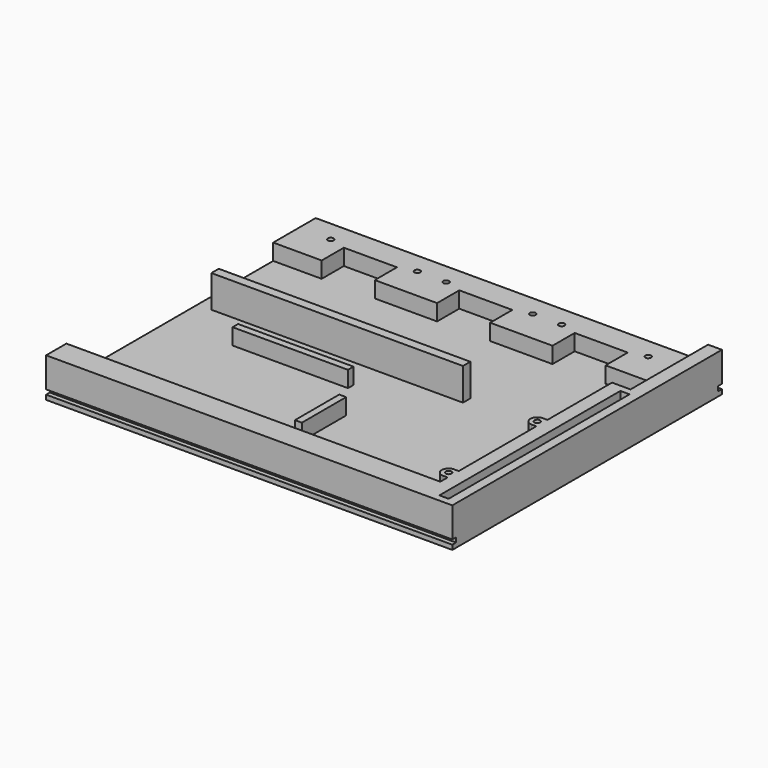
from build123d import *

# Parameters (mm, degrees)
F0_W      = 176
F0_H      = 146
F1_DEPTH  = 3
F2_W      = 50
F2_H      = 3
F2_W_2    = 3
F2_H_2    = 24
F2_W_3    = 109
F2_H_3    = 4
F2_R      = 1.25
F3_DEPTH  = 7
F3_FACE_W = 109
F3_FACE_H = 4
F4_R      = 1.25
F4_W      = 4
F4_H      = 98
F5_DEPTH  = 7
F6_W      = 2
F6_H      = 2
F7_DEPTH  = 176


# Not quite as in the source:
# - a feature names something its author has since deleted; it is built from what else it names


with BuildPart() as f1:
    # F0 (on Top) → F1 (new body)
    with BuildSketch(Plane.XY):
        with Locations((88, 73)):
            Rectangle(F0_W, F0_H)
    extrude(amount=F1_DEPTH)

    # F2 (on face) → F3 (join)
    with BuildSketch(Plane.XY.offset(3)):
        with Locations((53, 67.5)):
            Rectangle(F2_W, F2_H)
        with Locations((88.5, 38)):
            Rectangle(F2_W_2, F2_H_2)
        with Locations((60.5, 84)):
            Rectangle(F2_W_3, F2_H_3)
        with BuildLine():
            Line((0, 123), (6, 123))
            Line((6, 123), (21, 123))
            Line((21, 123), (21, 135))
            Line((21, 135), (44, 135))
            Line((44, 135), (44, 123))
            Line((44, 123), (71, 123))
            Line((71, 123), (71, 135))
            Line((71, 135), (94, 135))
            Line((94, 135), (94, 123))
            Line((94, 123), (121, 123))
            Line((121, 123), (121, 135))
            Line((121, 135), (144, 135))
            Line((144, 135), (144, 123))
            Line((144, 123), (170, 123))
            Line((170, 123), (170, 104))
            Line((170, 104), (162, 104))
            Line((162, 104), (162, 69))
            Line((162, 69), (160, 69))
            ThreePointArc((160, 69), (157, 66), (160, 63))
            Line((160, 63), (162, 63))
            Line((162, 63), (162, 21))
            Line((162, 21), (160, 21))
            ThreePointArc((160, 21), (157, 18), (160, 15))
            Line((160, 15), (162, 15))
            Line((162, 15), (162, 11))
            Line((162, 11), (0, 11))
            Line((0, 11), (0, 0))
            Line((0, 0), (176, 0))
            Line((176, 0), (176, 146))
            Line((176, 146), (0, 146))
            Line((0, 146), (0, 123))
        make_face()
        with Locations((13.75, 137)):
            Circle(F2_R, mode=Mode.SUBTRACT)
        with Locations((51.25, 137)):
            Circle(F2_R, mode=Mode.SUBTRACT)
        with Locations((63.75, 137)):
            Circle(F2_R, mode=Mode.SUBTRACT)
        with Locations((101.25, 137)):
            Circle(F2_R, mode=Mode.SUBTRACT)
        with Locations((113.75, 137)):
            Circle(F2_R, mode=Mode.SUBTRACT)
        with Locations((151.25, 137)):
            Circle(F2_R, mode=Mode.SUBTRACT)
    extrude(amount=F3_DEPTH)

    # F3_face (on face) + F4 (on face) → F5 (join)
    with BuildSketch(Plane(origin=(60.5, 84, 10), x_dir=(1, 0, 0), z_dir=(0, 0, 1))):
        Rectangle(F3_FACE_W, F3_FACE_H)
    with BuildSketch(Plane.XY.offset(10)):
        with BuildLine():
            Line((170, 146), (170, 123))
            Line((170, 123), (170, 104))
            Line((170, 104), (162, 104))
            Line((162, 104), (162, 69))
            Line((162, 69), (160, 69))
            ThreePointArc((160, 69), (157, 66), (160, 63))
            Line((160, 63), (162, 63))
            Line((162, 63), (162, 21))
            Line((162, 21), (160, 21))
            ThreePointArc((160, 21), (157, 18), (160, 15))
            Line((160, 15), (162, 15))
            Line((162, 15), (162, 11))
            Line((162, 11), (0, 11))
            Line((0, 11), (0, 0))
            Line((0, 0), (176, 0))
            Line((176, 0), (176, 146))
            Line((176, 146), (170, 146))
        make_face()
        with Locations((160, 18)):
            Circle(F4_R, mode=Mode.SUBTRACT)
        with Locations((170, 52)):
            Rectangle(F4_W, F4_H, mode=Mode.SUBTRACT)
        with Locations((160, 66)):
            Circle(F4_R, mode=Mode.SUBTRACT)
    extrude(amount=F5_DEPTH)

    # F6 (on face) → F7 (cut)
    with BuildSketch(Plane(origin=(0, 0, 0), x_dir=(0, -1, 0), z_dir=(-1, 0, 0))):
        with Locations((-145, 3)):
            Rectangle(F6_W, F6_H)
        with Locations((-1, 3)):
            Rectangle(F6_W, F6_H)
    extrude(amount=-F7_DEPTH, mode=Mode.SUBTRACT)


solid = f1.part
